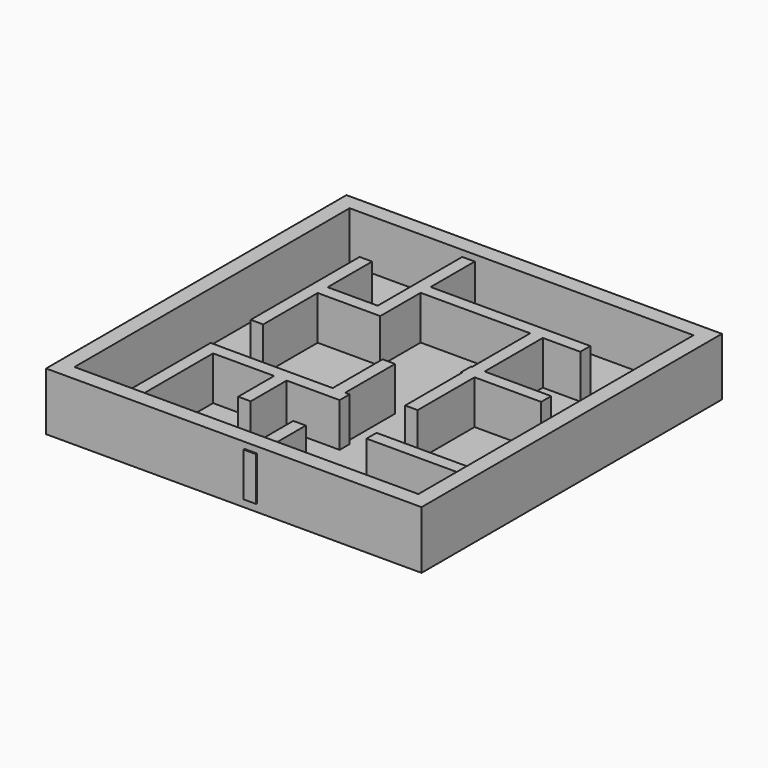
from build123d import *

# Parameters (mm, degrees)
F0_W      = 38.1
F0_H      = 38.1
F1_DEPTH  = 0.79375
F2_W      = 38.1
F2_H      = 38.1
F2_W_2    = 34.8996
F2_H_2    = 34.8996
F3_DEPTH  = 5.08
F4_W      = 1.27
F4_H      = 10.9915577808
F4_H_2    = 10.7192572
F5_DEPTH  = 4.445
F7_W      = 1.27
F7_H      = 6.305353716
F9_DEPTH  = 4.445
F8_W      = 1.27
F8_H      = 7.127109261
F8_H_2    = 15.866300866
F8_W_2    = 9.8573208662
F8_H_3    = 1.27
F10_DEPTH = 4.445
F11_W     = 8.128
F11_H     = 1.27
F12_DEPTH = 4.445


# Not quite as in the source:
# - a feature names something its author has since deleted; it is built from what else it names


with BuildPart() as f1:
    # F0 (on Top) → F1 (new body)
    with BuildSketch(Plane.XY):
        with Locations((0.9067468345, -3.6591270581)):
            Rectangle(F0_W, F0_H)
    extrude(amount=F1_DEPTH)

    # F2 (on face) → F3 (join)
    with BuildSketch(Plane.XY.offset(0.79375)):
        with Locations((0.9067468345, -3.6591270581)):
            Rectangle(F2_W, F2_H)
        with Locations((0.9067468345, -3.6591270581)):
            Rectangle(F2_W_2, F2_H_2, mode=Mode.SUBTRACT)
    extrude(amount=F3_DEPTH)

    # F4 (on face) → F5 (join)
    with BuildSketch(Plane.XY.offset(0.79375)):
        with Locations((-10.8280531655, -15.6836010049)):
            Rectangle(F4_W, F4_H)
        Polygon((-11.4630531655, -5.1078221145), (-10.1930531655, -5.1078221145), (-10.1930531655, 1.8014254137), (-10.1930531655, 3.0714254137), (-10.1930531655, 8.7106729419), (-11.4630531655, 8.7106729419), align=None)
        Polygon((-10.1930531655, 3.0714254137), (-10.1930531655, 1.8014254137), (-3.8430531655, 1.8014254137), (-3.8430531655, 3.0714254137), (-5.1130531655, 3.0714254137), align=None)
        with Locations((-4.4780531655, 8.4310540137)):
            Rectangle(F4_W, F4_H_2)
    extrude(amount=F5_DEPTH)

    # F7 (on face) → F9 (join)
    with BuildSketch(Plane.XY.offset(0.79375)):
        Polygon((2.6555440854, -10.197567645), (-10.6428060681, -10.197567645), (-10.6428060681, -11.467567645), (-3.9936309913, -11.467567645), (-3.9936309913, -16.0289270581), (-2.7236309913, -16.0289270581), (-2.7236309913, -11.467567645), (2.6555440854, -11.467567645), align=None)
        with Locations((2.6458618774, -19.700244503)):
            Rectangle(F7_W, F7_H)
    extrude(amount=F9_DEPTH)

    # F8 (on face) → F10 (join)
    with BuildSketch(Plane.XY.offset(0.79375)):
        with Locations((1.5678320881, -7.4372278345)):
            Rectangle(F8_W, F8_H)
        Polygon((12.3628337599, 8.1913313339), (-4.464668509, 8.1913313339), (-4.464668509, 6.9213313339), (7.2828320881, 6.9213313339), (8.5528320881, 6.9213313339), (12.3628337599, 6.9213313339), align=None)
        with Locations((7.9178320881, -1.0118190991)):
            Rectangle(F8_W, F8_H_2)
        with Locations((13.370096651, -14.6599695321)):
            Rectangle(F8_W_2, F8_H_3)
    extrude(amount=F10_DEPTH)

    # F11 (on face) → F12 (join)
    with BuildSketch(Plane.XY.offset(0.79375)):
        with Locations((11.246104741, -1.0928286647)):
            Rectangle(F11_W, F11_H)
    extrude(amount=F12_DEPTH)


solid = f1.part
